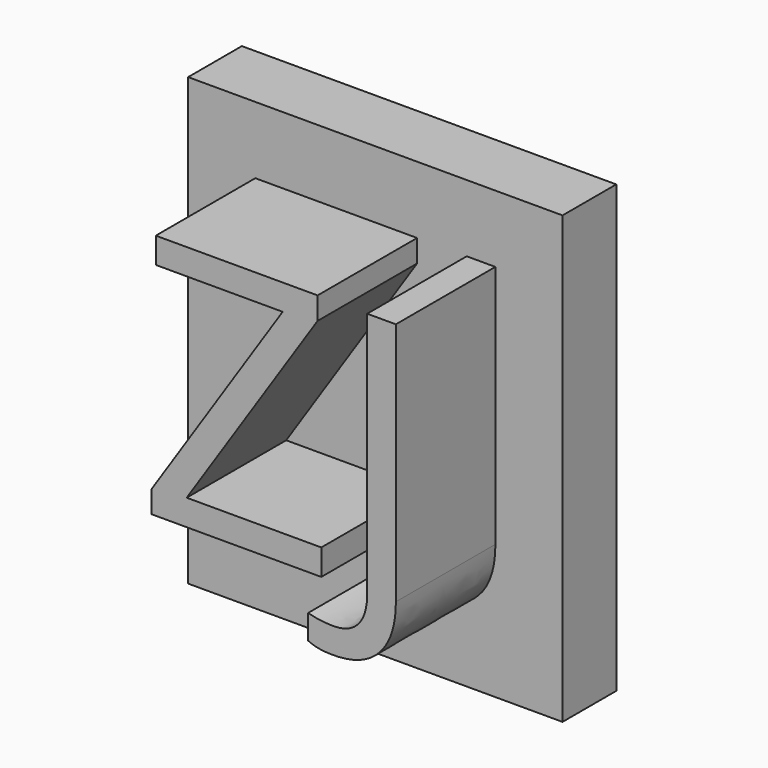
from build123d import *

# Parameters (mm, degrees)
F1_TEXT_SIZE = 35.2777777778
F2_DEPTH     = 12.7
F4_W         = 38.2285434028
F4_H         = 45.5321458333
F5_DEPTH     = 6.858


# Not quite as in the source:
# - a variable given as a bare number and used for a length is read in inches; the dataset says mm whatever the document's units were
# - Text() gives the source's letters only with a copy of the font that has no kerning and outlines rounded to 1/6400 em; it was checked with that copy


with BuildPart() as f2:
    # F1 (on Front) → F2 (new body)
    with BuildSketch(Plane.XZ):
        with Locations((-15.4695156792, -13.7332208696)):
            Text('ZJ', F1_TEXT_SIZE, font='Open Sans', text_align=(TextAlign.LEFT, TextAlign.BOTTOM))
    extrude(amount=F2_DEPTH)

    # F4 (on Front) → F5 (join)
    with BuildSketch(Plane.XZ):
        with Locations((-1.3887214083, -4.4562677446)):
            Rectangle(F4_W, F4_H)
    extrude(amount=-F5_DEPTH)


solid = f2.part
